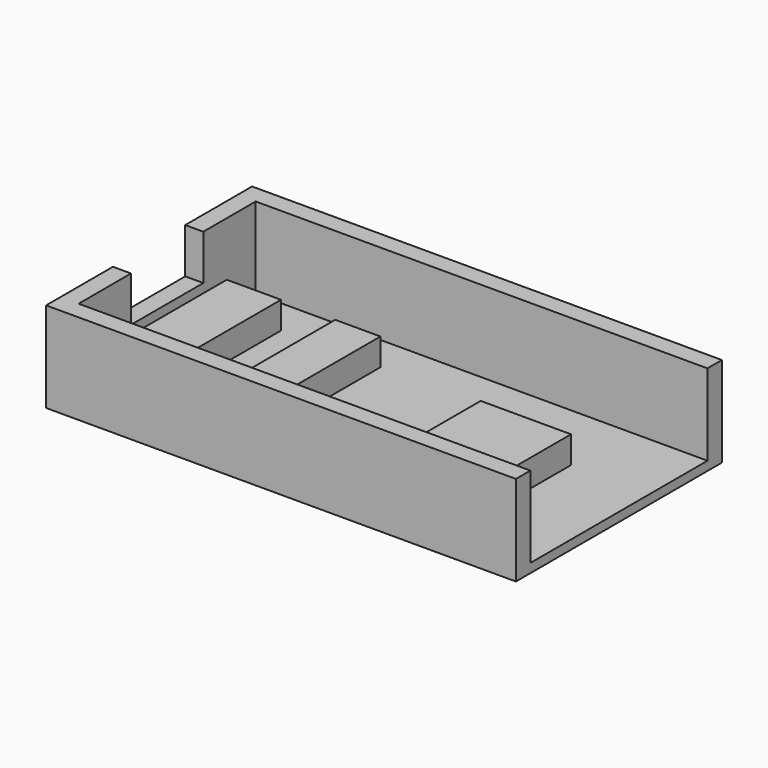
from build123d import *

# Parameters (mm, degrees)
F0_W     = 5
F0_H     = 16.5
F0_W_2   = 10
F0_H_2   = 8.5
F1_DEPTH = 1
F2_DEPTH = 4
F0_W_3   = 2
F0_H_3   = 10
F3_DEPTH = 5
F0_W_4   = 50
F0_H_4   = 2
F4_DEPTH = 10


# Not quite as in the source:
# - a feature names something its author has since deleted; it is built from what else it names


with BuildPart() as f1:
    # F0 (on Top) → F1 (new body)
    with BuildSketch(Plane.XY):
        Polygon((2, 6), (2, 2), (52, 2), (52, 6), (52, 26.5), (2, 26.5), (2, 22.5), (8, 22.5), (8, 6), align=None)
        with Locations((16.5, 14.25)):
            Rectangle(F0_W, F0_H, mode=Mode.SUBTRACT)
        with Locations((38.3, 14.25)):
            Rectangle(F0_W_2, F0_H_2, mode=Mode.SUBTRACT)
    extrude(amount=F1_DEPTH)

    # F0 (on Top) → F2 (join)
    with BuildSketch(Plane.XY):
        Polygon((2, 19.25), (2, 9.25), (2, 6), (8, 6), (8, 22.5), (2, 22.5), align=None)
        with Locations((16.5, 14.25)):
            Rectangle(F0_W, F0_H)
        with Locations((38.3, 14.25)):
            Rectangle(F0_W_2, F0_H_2)
    extrude(amount=F2_DEPTH)

    # F0 (on Top) → F3 (join)
    with BuildSketch(Plane.XY):
        with Locations((1, 14.25)):
            Rectangle(F0_W_3, F0_H_3)
    extrude(amount=F3_DEPTH)

    # F0 (on Top) → F4 (join)
    with BuildSketch(Plane.XY):
        with Locations((27, 27.5)):
            Rectangle(F0_W_4, F0_H_4)
        Polygon((0, 28.5), (0, 19.25), (2, 19.25), (2, 22.5), (2, 26.5), (2, 28.5), align=None)
        Polygon((0, 9.25), (0, 0), (2, 0), (2, 2), (2, 6), (2, 9.25), align=None)
        with Locations((27, 1)):
            Rectangle(F0_W_4, F0_H_4)
    extrude(amount=F4_DEPTH)


solid = f1.part
